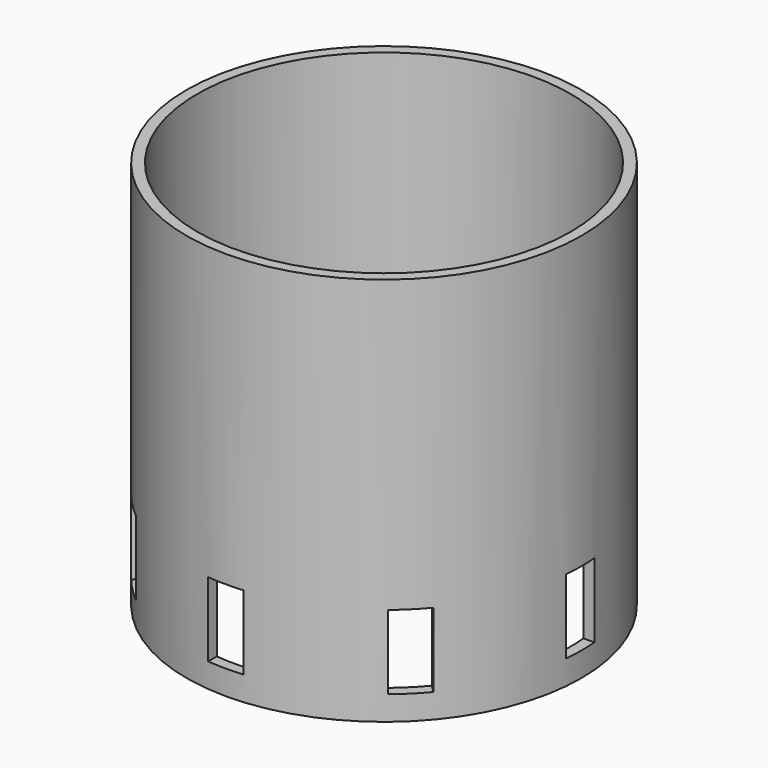
from build123d import *

# Parameters (mm, degrees)
F0_R            = 51.5338548396
F0_R_2          = 48.7228938758
F1_DEPTH        = 101.6
F2_W            = 9.2484680936
F2_H            = 19.3572561257
F3_DEPTH        = 127
F3_COPIES_COUNT = 8


# Not quite as in the source:
# - a pattern or mirror of a feature is missing from the dataset's text; its kind, count and spacing are read off the source's solid


with BuildPart() as f1:
    # F0 (on Top) → F1 (new body)
    with BuildSketch(Plane.XY):
        Circle(F0_R)
        Circle(F0_R_2, mode=Mode.SUBTRACT)
    extrude(amount=F1_DEPTH)

    # F2 (on Front) → F3 (cut)
    with BuildSketch(Plane.XZ):
        with Locations((0.215081498, 16.0337483976)):
            Rectangle(F2_W, F2_H)
    f3 = extrude(amount=-F3_DEPTH, mode=Mode.SUBTRACT)

    # F3_copies: F3 ×8 about axis
    f3_copies_axis = Axis((0, 0, 0), (0, 0, 1))
    for i in range(1, F3_COPIES_COUNT):
        add(f3.rotate(f3_copies_axis, i * 360 / F3_COPIES_COUNT), mode=Mode.SUBTRACT)


solid = f1.part
